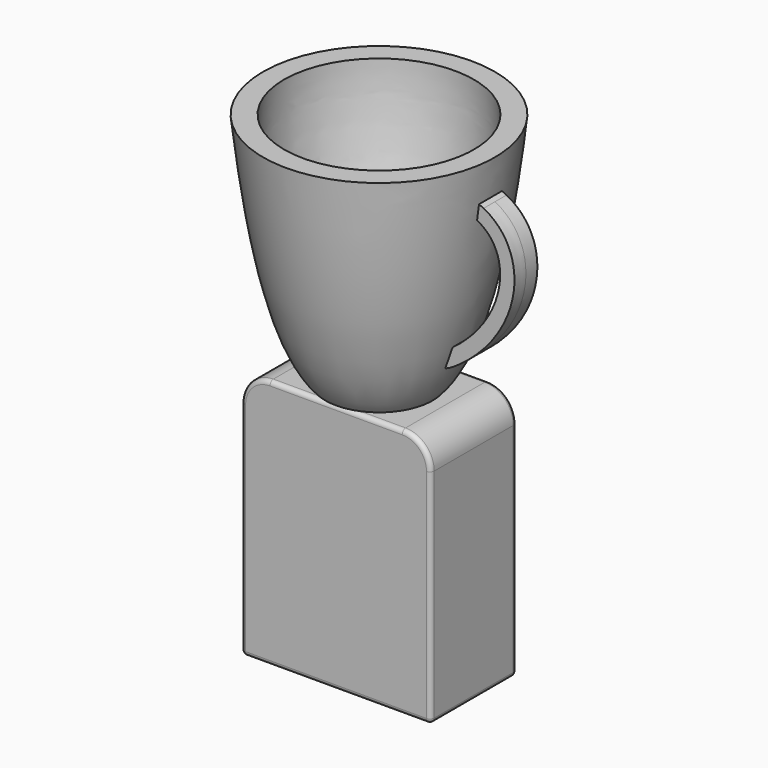
from build123d import *

# Parameters (mm, degrees)
F1_DEPTH = 9.525
F2_R     = 0.762
F4_DEPTH = 2.54
F5_W     = 10.3596793488
F5_H     = 7.399763912
F6_DEPTH = 1.524


# Not quite as in the source:
# - the dataset's text gives a spline's control points without its knots; the knots are read off the source's solid


with BuildPart() as f1:
    # F0 (on Front) → F1 (new body, symmetric)
    with BuildSketch(Plane.XZ):
        with BuildLine():
            ThreePointArc((16.8140027672, -5.08), (15.3261052156, -1.4878975516), (11.7340027672, 0))
            Line((11.7340027672, 0), (9.5236673951, 0))
            Line((9.5236673951, 0), (0, 0))
            Line((0, 0), (-7.2401063517, 0))
            Line((-7.2401063517, 0), (-9.5236673951, 0))
            Line((-9.5236673951, 0), (-11.7340027672, 0))
            ThreePointArc((-11.7340027672, 0), (-15.3261052156, -1.4878975516), (-16.8140027672, -5.08))
            Line((-16.8140027672, -5.08), (-16.8140027672, -44.433273375))
            Line((-16.8140027672, -44.433273375), (16.8140027672, -44.433273375))
            Line((16.8140027672, -44.433273375), (16.8140027672, -5.08))
        make_face()
    extrude(amount=F1_DEPTH, both=True)

    # F2
    f2_edges = [f1.edges().sort_by_distance(p)[0] for p in [
        (0, -9.525, 0),
        (16.814003, -9.525, -24.756637),
        (15.326105, -9.525, -1.487898),
        (15.326105, 9.525, -1.487898),
        (0, 9.525, 0),
        (16.814003, 9.525, -24.756637),
        (-15.326105, 9.525, -1.487898),
        (-16.814003, 9.525, -24.756637),
        (0, 9.525, -44.433273),
        (-15.326105, -9.525, -1.487898),
        (-16.814003, -9.525, -24.756637),
        (0, -9.525, -44.433273),
        (-16.814003, 0, -5.08),
        (-16.814003, 0, -44.433273),
        (16.814003, 0, -5.08),
        (16.814003, 0, -44.433273),
    ]]
    fillet(f2_edges, radius=F2_R)

    # F5 (on face) → F6 (join)
    with BuildSketch(Plane(origin=(-16.8140027672, 0, 0), x_dir=(0, -1, 0), z_dir=(-1, 0, 0))):
        with Locations((0, -22.6617902517)):
            Rectangle(F5_W, F5_H)
    extrude(amount=F6_DEPTH)


with BuildPart() as f3:
    # F0 (on Front) → F3 (revolve)
    with BuildSketch(Plane.XZ):
        with BuildLine():
            Line((-9.5236673951, 0), (-7.2401063517, 0))
            add(Edge.make_bspline(
                [(-16.8360508978, 41.5870919824), (-16.8553277932, 38.8545802624), (-16.5581952608, 31.2683940077), (-12.3689733446, 11.3153951243), (-7.2401063517, 0)],
                knots=[0, 0, 0, 0, 0.348881703, 1, 1, 1, 1], degree=3))
            Line((-16.8360508978, 41.5870919824), (-20.5721743405, 41.5870919824))
            add(Edge.make_bspline(
                [(-20.5721743405, 41.5870919824), (-19.4350704551, 31.8282805383), (-16.7806390673, 7.7172145247), (-9.5236673951, 0)],
                knots=[0, 0, 0, 0, 43.0297074737, 43.0297074737, 43.0297074737, 43.0297074737], degree=3))
        make_face()
    revolve(axis=Axis((0, 0, 20.7935459912), (0, 0, 1)))


with BuildPart() as f4:
    # F0 (on Front) → F4 (new body, symmetric)
    with BuildSketch(Plane.XZ):
        with BuildLine():
            add(Edge.make_bspline(
                [(15.0883483115, 11.1491326454), (14.6839512093, 9.8533166215), (14.2523389086, 8.6080504568), (13.7915127177, 7.4332523839)],
                knots=[29.5353429201, 29.5353429201, 29.5353429201, 29.5353429201, 33.2585908266, 33.2585908266, 33.2585908266, 33.2585908266], degree=3))
            add(Edge.make_bspline(
                [(16.5973321119, 9.1059567131), (15.7718844712, 8.504178375), (14.8418424651, 7.8182732686), (13.7915127177, 7.4332523839)],
                knots=[0, 0, 0, 0, 3.2665826556, 3.2665826556, 3.2665826556, 3.2665826556], degree=3))
            add(Edge.make_bspline(
                [(20.5968842238, 34.6659384297), (21.6884105691, 34.104490474), (23.1260600945, 33.0034985903), (24.526596028, 31.141826143), (25.5668613568, 29.0824519601), (26.1939854164, 26.2505211334), (25.9764658619, 22.6813598881), (24.8851440982, 19.0678312081), (22.3274130345, 14.3300367076), (19.2019247954, 11.0295738153), (16.5973321119, 9.1059567131)],
                knots=[0, 0, 0, 0, 0.125, 0.1875, 0.25, 0.375, 0.5, 0.625, 0.75, 1, 1, 1, 1], degree=3))
            Line((20.5968842238, 34.6659384297), (19.784617424, 35.0388268786))
            add(Edge.make_bspline(
                [(19.784617424, 35.0388268786), (19.6759864871, 34.1916570064), (19.5597008725, 33.3121636908), (19.4350704551, 32.4072244666)],
                knots=[7.8099300685, 7.8099300685, 7.8099300685, 7.8099300685, 10.4219868825, 10.4219868825, 10.4219868825, 10.4219868825], degree=3))
            add(Edge.make_bspline(
                [(19.4350704551, 32.4072244666), (26.1015295982, 28.9782006294), (24.6091987938, 18.1807391346), (15.0883483115, 11.1491326454)],
                knots=[0, 0, 0, 0, 21.6979367976, 21.6979367976, 21.6979367976, 21.6979367976], degree=3))
        make_face()
    extrude(amount=F4_DEPTH, both=True)


solid = Compound([f1.part, f3.part, f4.part])
